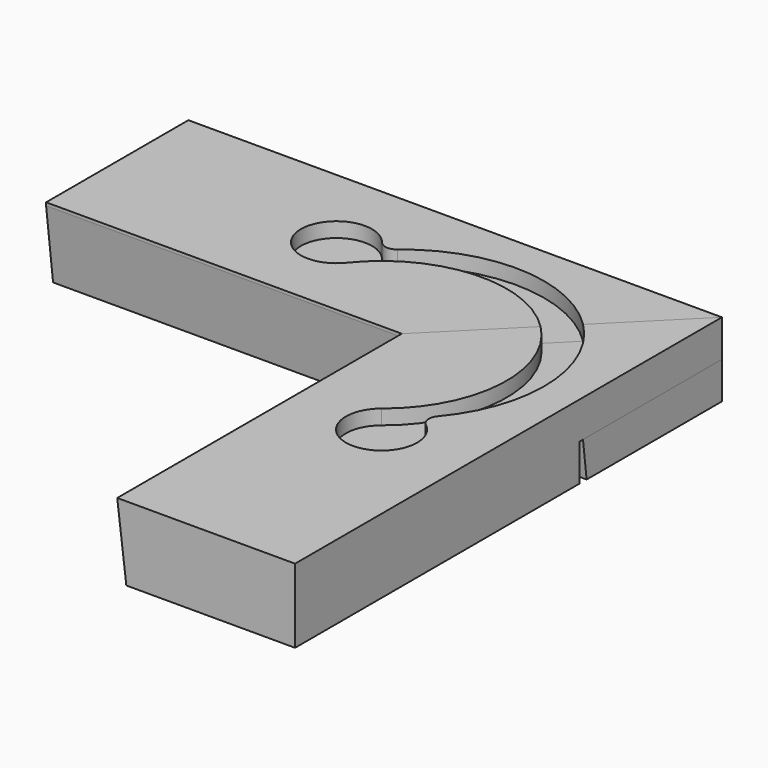
from build123d import *

# Parameters (mm, degrees)
F2_DEPTH     = 12.5
F3_W         = 180
F3_H         = 60
F4_DEPTH     = 12.5
F5_SIZE2     = 2.9468294617
F5_SIZE      = 24
F7_DEPTH     = 12.5
F8_W         = 60
F8_H         = 120
F9_DEPTH     = 12.5
F10_T1_DEPTH = 249.96415925
F13_DEPTH    = 5


# Not quite as in the source:
# - a fillet or chamfer that OpenCascade refuses, or shapes differently, is made with other operations: its cross-section is extruded or revolved along the edge and cut away or added


with BuildPart() as f2:
    # F1 (on Top) → F2 (new body)
    with BuildSketch(Plane.XY):
        Polygon((-120, 0), (0, 0), (12.6794919243, 12.6794919243), (47.3205080757, 47.3205080757), (60, 60), (-120, 60), align=None)
    extrude(amount=F2_DEPTH)

    # F3 (on Top) → F4 (join)
    with BuildSketch(Plane.XY):
        with Locations((-30, 30)):
            Rectangle(F3_W, F3_H)
    extrude(amount=-F4_DEPTH)

    # F5
    f5_edges = [f2.edges().sort_by_distance(p)[0] for p in [
        (-30, 0, -12.5),
    ]]
    f5_side = f2.faces().sort_by_distance((-42, 0, -1.25))[0]
    chamfer(f5_edges, length=F5_SIZE, length2=F5_SIZE2, reference=f5_side)


with BuildPart() as f7:
    # F6 (on Top) → F7 (new body)
    with BuildSketch(Plane.XY):
        Polygon((60, -120), (60, 60), (47.3205080757, 47.3205080757), (12.6794919243, 12.6794919243), (0, 0), (0, -120), align=None)
    extrude(amount=F7_DEPTH)

    # F8 (on face) → F9 (join)
    with BuildSketch(Plane(origin=(0, 0, 0), x_dir=(1, 0, 0), z_dir=(0, 0, -1))):
        with Locations((30, 60)):
            Rectangle(F8_W, F8_H)
    extrude(amount=F9_DEPTH)

    # F10: chamfer of 25 x 3.0696140226 on 1 edges, made by hand

    # F10_s2 → F10_t1 (cut)
    with BuildSketch(Plane.XZ.offset(-64.982079625)):
        Polygon((3.0696140226, -12.5), (0, 12.5), (0, -12.5), align=None)
    extrude(amount=F10_T1_DEPTH, mode=Mode.SUBTRACT)


with BuildPart() as f13_tool:
    # F12 (on plane+point) → F13 (new body)
    with BuildSketch(Plane.XY.offset(12.5)):
        with BuildLine():
            ThreePointArc((37.4123746331, -36.5984442616), (35.9045811532, -33.8661359121), (36.8184902357, -30.8822256783))
            ThreePointArc((36.8184902357, -30.8822256783), (33.9802375365, 33.9802375365), (-30.8822256783, 36.8184902357))
            ThreePointArc((-30.8822256783, 36.8184902357), (-33.8661359121, 35.9045811532), (-36.5984442616, 37.4123746331))
            ThreePointArc((-36.5984442616, 37.4123746331), (-58.0353381129, 30.0469938735), (-36.6567893055, 22.5139398702))
            ThreePointArc((-36.6567893055, 22.5139398702), (26.0197624635, 26.0197624635), (22.5139398702, -36.6567893055))
            ThreePointArc((22.5139398702, -36.6567893055), (30.0469938735, -58.0353381129), (37.4123746331, -36.5984442616))
        make_face()
    extrude(amount=-F13_DEPTH)


with BuildPart() as f2_1:
    add(f2.part)

    # F13: cut by f13_tool
    add(f13_tool.part, mode=Mode.SUBTRACT)


with BuildPart() as f7_1:
    add(f7.part)

    # F13: cut by f13_tool
    add(f13_tool.part, mode=Mode.SUBTRACT)


solid = Compound([f2_1.part, f7_1.part])
